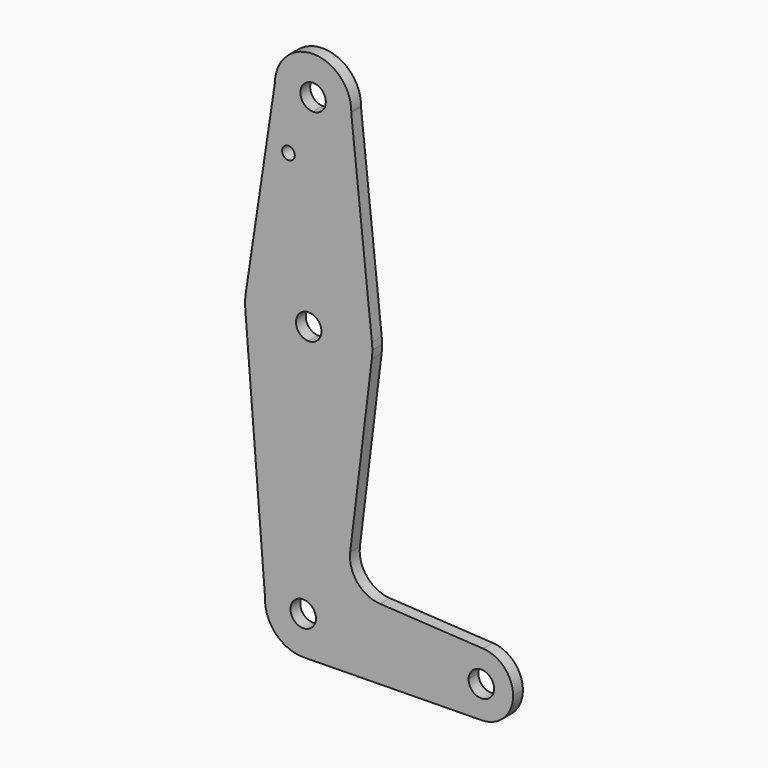
from build123d import *

# Parameters (mm, degrees)
F0_R     = 1.5875
F1_DEPTH = 3.048


# Not quite as in the source:
# - ends of sketch curves that miss each other by under 0.0002 mm in the source are joined


with BuildPart() as f1:
    # F0 (on Front) → F1 (new body)
    with BuildSketch(Plane.XZ):
        with BuildLine():
            Line((9.5227532787, -40.8667611849), (3.1742510929, -40.7288481794))
            ThreePointArc((3.1742510929, -40.7288481794), (-2.2931551214, -42.8558116635), (0.0685547428, -37.4856318814))
            Line((0.0685547428, -37.4856318814), (0.2056642284, -31.1371122911))
            ThreePointArc((0.2056642284, -31.1371122911), (-6.5169022357, -33.713265859), (-9.5165120399, -40.2578673054))
            ThreePointArc((-9.5165120399, -40.2578673054), (-6.8758602056, -47.2514143711), (0, -50.1848916766))
            Line((0, -50.1848916766), (0.266136468, -50.1811729129))
            ThreePointArc((0.266136468, -50.1811729129), (6.7561199721, -47.3740906551), (9.5227532787, -40.8667611849))
        make_face()
        with BuildLine():
            ThreePointArc((9.525, -40.6598916766), (9.5244383031, -40.7633325307), (9.5227532787, -40.8667611849))
            Line((9.5227532787, -40.8667611849), (36.5143722678, -41.4531192251))
            ThreePointArc((36.5143722678, -41.4531192251), (39.0634111277, -35.7955390781), (44.9045471293, -33.7010361679))
            Line((44.9045471293, -33.7010361679), (19.1536412274, -32.2239665364))
            ThreePointArc((19.1536412274, -32.2239665364), (13.5071817385, -29.3833337913), (11.7175692398, -23.3212395774))
            Line((11.7175692398, -23.3212395774), (17.1169295277, 20.8061344164))
            ThreePointArc((17.1169295277, 20.8061344164), (11.7244811987, 10.8044243048), (1.0286415004, 6.9688386539))
            Line((1.0286415004, 6.9688386539), (0.2056642284, -31.1371122911))
            ThreePointArc((0.2056642284, -31.1371122911), (6.8075170501, -33.9978096738), (9.525, -40.6598916766))
        make_face()
        with BuildLine():
            Line((36.5143722678, -41.4531192251), (9.5227532787, -40.8667611849))
            ThreePointArc((9.5227532787, -40.8667611849), (6.7561199721, -47.3740906551), (0.266136468, -50.1811729129))
            Line((0.266136468, -50.1811729129), (44.5609010201, -49.5622357019))
            ThreePointArc((44.5609010201, -49.5622357019), (38.8156384977, -47.216384896), (36.5143722678, -41.4531192251))
        make_face()
        with BuildLine():
            ThreePointArc((-9.5165120399, -40.2578673054), (-6.5169022357, -33.713265859), (0.2056642284, -31.1371122911))
            Line((0.2056642284, -31.1371122911), (1.0286415004, 6.9688386539))
            ThreePointArc((1.0286415004, 6.9688386539), (-9.5225283922, 11.2941952389), (-14.4519047173, 21.5770520761))
            Line((-14.4519047173, 21.5770520761), (-9.5165120399, -40.2578673054))
        make_face()
        with BuildLine():
            ThreePointArc((44.9045471293, -33.7010361679), (39.0634111277, -35.7955390781), (36.5143722678, -41.4531192251))
            ThreePointArc((36.5143722678, -41.4531192251), (38.8156384977, -47.216384896), (44.5609010201, -49.5622357019))
            ThreePointArc((44.5609010201, -49.5622357019), (50.1017334994, -47.1988232045), (52.3875, -41.6255104821))
            ThreePointArc((52.3875, -41.6255104821), (50.221129616, -36.1759261672), (44.9045471293, -33.7010361679))
        make_face()
        with BuildLine():
            ThreePointArc((47.625, -41.6255104821), (44.4155197153, -44.8003232498), (41.2757489071, -41.5565539793))
            ThreePointArc((41.2757489071, -41.5565539793), (44.4844802847, -38.4506977144), (47.625, -41.6255104821))
        make_face(mode=Mode.SUBTRACT)
        with BuildLine():
            ThreePointArc((0, -50.1848916766), (0.1330812241, -50.1839619403), (0.266136468, -50.1811729129))
            Line((0.266136468, -50.1811729129), (0, -50.1848916766))
        make_face()
        with BuildLine():
            Line((1.3028604766, 19.6658780657), (1.0286415004, 6.9688386539))
            ThreePointArc((1.0286415004, 6.9688386539), (11.7244811987, 10.8044243048), (17.1169295277, 20.8061344164))
            ThreePointArc((17.1169295277, 20.8061344164), (17.2150257343, 21.821019398), (17.2477694947, 22.8401083234))
            ThreePointArc((17.2477694947, 22.8401083234), (17.2256547172, 23.6777568916), (17.1593719988, 24.5130716756))
            ThreePointArc((17.1593719988, 24.5130716756), (12.1164496714, 34.5272363394), (1.714188926, 38.71143649))
            Line((1.714188926, 38.71143649), (1.4399699498, 26.0143970782))
            ThreePointArc((1.4399699498, 26.0143970782), (3.6414680693, 25.0612863392), (4.5477694947, 22.8401083234))
            ThreePointArc((4.5477694947, 22.8401083234), (3.5929793798, 20.5704623012), (1.3028604766, 19.6658780657))
        make_face()
        with BuildLine():
            ThreePointArc((-14.4519047173, 21.5770520761), (-9.5225283922, 11.2941952389), (1.0286415004, 6.9688386539))
            Line((1.0286415004, 6.9688386539), (1.3028604766, 19.6658780657))
            ThreePointArc((1.3028604766, 19.6658780657), (-1.8014903005, 22.9086630662), (1.4399699498, 26.0143970782))
            Line((1.4399699498, 26.0143970782), (1.714188926, 38.71143649))
            ThreePointArc((1.714188926, 38.71143649), (-8.8575904586, 34.9791099391), (-14.3269783089, 25.1924569167))
            ThreePointArc((-14.3269783089, 25.1924569167), (-14.4927618199, 23.388324618), (-14.4519047173, 21.5770520761))
        make_face()
        with BuildLine():
            Line((-7.0564734592, 73.7163418848), (-14.3269783089, 25.1924569167))
            ThreePointArc((-14.3269783089, 25.1924569167), (-8.8575904586, 34.9791099391), (1.714188926, 38.71143649))
            Line((1.714188926, 38.71143649), (2.2623065092, 64.0906813969))
            ThreePointArc((2.2623065092, 64.0906813969), (-4.375426743, 66.9882410244), (-7.0564734592, 73.7163418848))
        make_face()
        with Locations((-3.6854336504, 59.3653083234)):
            Circle(F0_R, mode=Mode.SUBTRACT)
        with BuildLine():
            Line((2.2623065092, 64.0906813969), (1.714188926, 38.71143649))
            ThreePointArc((1.714188926, 38.71143649), (12.1164496714, 34.5272363394), (17.1593719988, 24.5130716756))
            Line((17.1593719988, 24.5130716756), (11.9881470583, 73.3103585299))
            ThreePointArc((11.9881470583, 73.3103585299), (9.0208819611, 66.700792671), (2.2623065092, 64.0906813969))
        make_face()
        with BuildLine():
            ThreePointArc((11.9929709084, 73.6134609496), (2.5194119609, 83.1383222076), (-7.0564737935, 73.7163418884))
            ThreePointArc((-7.0564737935, 73.7163418884), (-4.375426743, 66.9882410244), (2.2623065092, 64.0906813969))
            ThreePointArc((2.2623065092, 64.0906813969), (9.0208819611, 66.700792671), (11.9881470583, 73.3103585299))
            ThreePointArc((11.9881470583, 73.3103585299), (11.9917648696, 73.4618905482), (11.9929709084, 73.6134609496))
        make_face()
        with BuildLine():
            ThreePointArc((5.6429707413, 73.6134609496), (4.6886647422, 71.3442885995), (2.3994159985, 70.4392011544))
            ThreePointArc((2.3994159985, 70.4392011544), (0.2472767404, 75.8826332996), (5.6429707413, 73.6134609496))
        make_face(mode=Mode.SUBTRACT)
        with BuildLine():
            ThreePointArc((3.175, -40.6598916766), (3.1748127677, -40.6943719613), (3.1742510929, -40.7288481794))
            Line((3.1742510929, -40.7288481794), (9.5227532787, -40.8667611849))
            ThreePointArc((9.5227532787, -40.8667611849), (9.5244383031, -40.7633325307), (9.525, -40.6598916766))
            ThreePointArc((9.525, -40.6598916766), (6.8075170501, -33.9978096738), (0.2056642284, -31.1371122911))
            Line((0.2056642284, -31.1371122911), (0.0685547428, -37.4856318814))
            ThreePointArc((0.0685547428, -37.4856318814), (2.26917235, -38.4391976756), (3.175, -40.6598916766))
        make_face()
    extrude(amount=F1_DEPTH)


solid = f1.part
